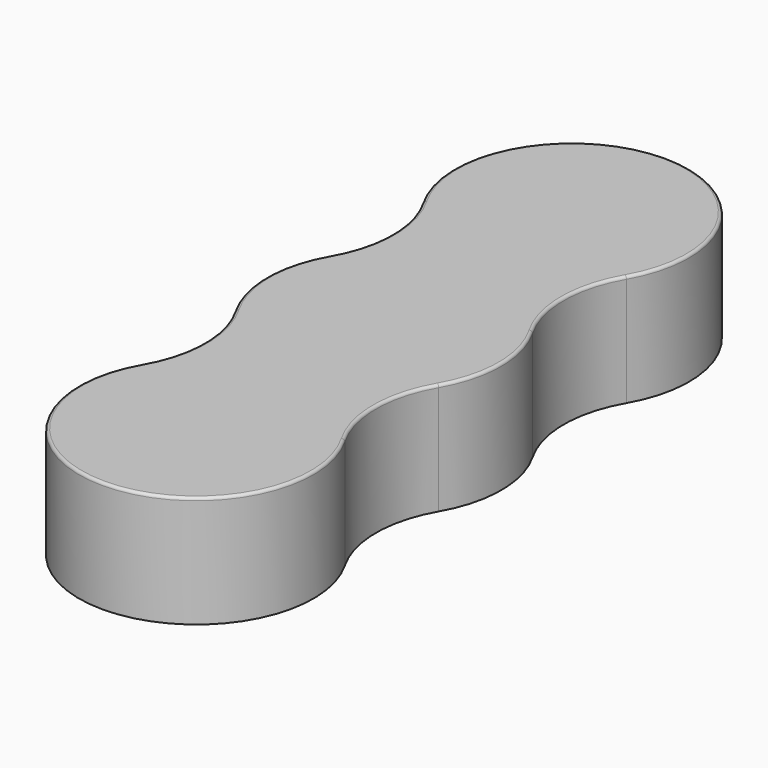
from build123d import *

# Parameters (mm, degrees)
F3_R     = 7.9
F4_DEPTH = 20
F5_DEPTH = 10
F6_R     = 0.5


# Not quite as in the source:
# - a feature names something its author has since deleted; it is built from what else it names


with BuildPart() as f4:
    # F3 (on Top) → F4 (new body)
    with BuildSketch(Plane.XY):
        with BuildLine():
            ThreePointArc((18.1865334795, 10.5), (15.3730669589, 21), (18.1865334795, 31.5))
            ThreePointArc((18.1865334795, 31.5), (21, 42), (18.1865334795, 52.5))
            ThreePointArc((18.1865334795, 52.5), (15.3730669589, 63), (18.1865334795, 73.5))
            ThreePointArc((18.1865334795, 73.5), (0, 105), (-18.1865334795, 73.5))
            ThreePointArc((-18.1865334795, 73.5), (-15.3730669589, 63), (-18.1865334795, 52.5))
            ThreePointArc((-18.1865334795, 52.5), (-21, 42), (-18.1865334795, 31.5))
            ThreePointArc((-18.1865334795, 31.5), (-15.3730669589, 21), (-18.1865334795, 10.5))
            ThreePointArc((-18.1865334795, 10.5), (0, -21), (18.1865334795, 10.5))
        make_face()
        Circle(F3_R, mode=Mode.SUBTRACT)
        with Locations((0, 42)):
            Circle(F3_R, mode=Mode.SUBTRACT)
        with Locations((0, 84)):
            Circle(F3_R, mode=Mode.SUBTRACT)
        with Locations((0, 42)):
            Circle(F3_R)
        Circle(F3_R)
        with Locations((0, 84)):
            Circle(F3_R)
    extrude(amount=F4_DEPTH)

    # F3 (on Top) → F5 (cut)
    with BuildSketch(Plane.XY):
        with Locations((0, 42)):
            Circle(F3_R)
        Circle(F3_R)
        with Locations((0, 84)):
            Circle(F3_R)
    extrude(amount=F5_DEPTH, mode=Mode.SUBTRACT)

    # F6
    f6_edges = [f4.edges().sort_by_distance(p)[0] for p in [
        (-7.9, 42, 0),
        (-7.9, 42, 10),
        (-7.9, 0, 0),
        (-7.9, 0, 10),
        (21, 42, 20),
        (-7.9, 84, 10),
        (-7.9, 84, 0),
        (15.373067, 21, 20),
        (0, -21, 20),
        (15.373067, 63, 20),
        (0, 105, 20),
        (-15.373067, 63, 20),
        (-21, 42, 20),
        (-15.373067, 21, 20),
    ]]
    fillet(f6_edges, radius=F6_R)


solid = f4.part
